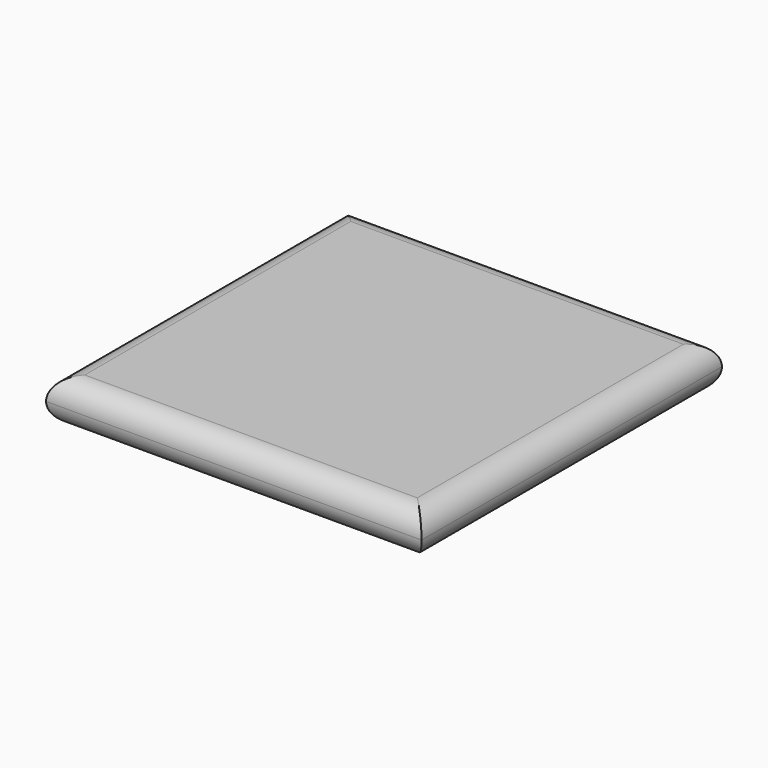
from build123d import *

# Parameters (mm, degrees)
F0_W     = 70
F0_H     = 70
F1_DEPTH = 8
F2_R     = 3.99999


# Not quite as in the source:
# - a fillet or chamfer is up to 0.001 mm smaller than in the source, because OpenCascade refuses the exact size


with BuildPart() as f1:
    # F0 (on Top) → F1 (new body)
    with BuildSketch(Plane.XY):
        Rectangle(F0_W, F0_H)
    extrude(amount=F1_DEPTH)

    # F2 (radius 4 in the source; OpenCascade refuses exactly that, so slightly less here)
    f2_edges = [f1.edges().sort_by_distance(p)[0] for p in [
        (0, -35, 8),
        (35, 0, 8),
        (0, 35, 8),
        (-35, 0, 8),
        (0, 35, 0),
        (-35, 0, 0),
        (0, -35, 0),
        (35, 0, 0),
    ]]
    fillet(f2_edges, radius=F2_R)


solid = f1.part
